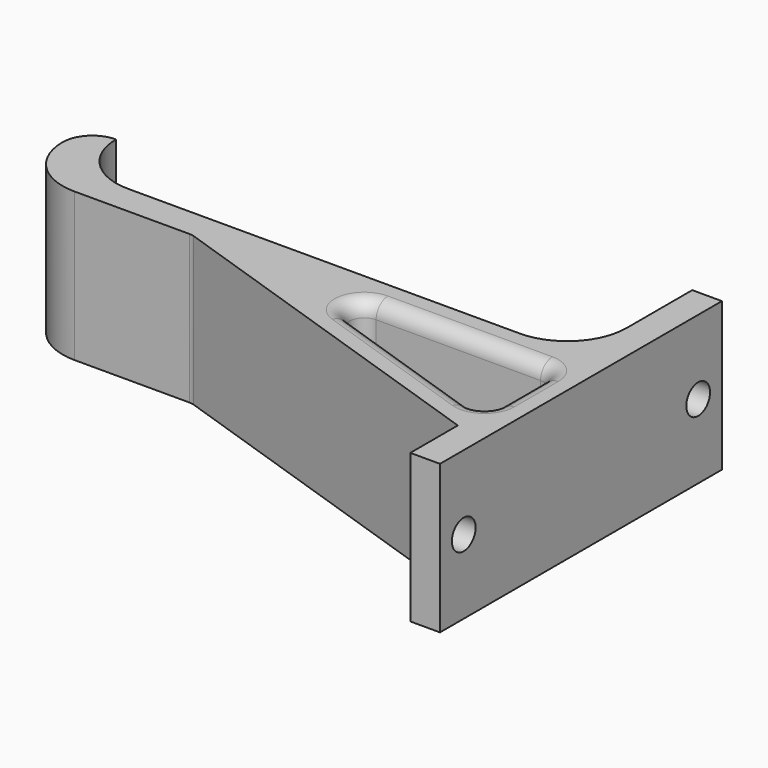
from build123d import *

# Parameters (mm, degrees)
F1_DEPTH = 25
F2_R     = 2.5
F3_DEPTH = 25
F4_R     = 4.99999
F5_F1_R  = 2.5
F5_F2_R  = 2.5
F5_F3_R  = 2.5


# Not quite as in the source:
# - a fillet or chamfer is up to 0.001 mm smaller than in the source, because OpenCascade refuses the exact size
# - a feature names something its author has since deleted; it is built from what else it names


with BuildPart() as f1:
    # F0 (on Top) → F1 (new body)
    with BuildSketch(Plane.XY):
        with BuildLine():
            ThreePointArc((11.9032669473, 15), (8.9743347592, 7.9289321881), (1.9032669473, 5))
            Line((1.9032669473, 5), (-64.0967330527, 5))
            ThreePointArc((-64.0967330527, 5), (-71.1678008646, 7.9289321881), (-74.0967330527, 15))
            Line((-74.0967330527, 15), (-79.0967330527, 15))
            Line((-79.0967330527, 15), (-79.0967330527, 10))
            ThreePointArc((-79.0967330527, 10), (-76.1678008646, 2.9289321881), (-69.0967330527, 0))
            Line((-69.0967330527, 0), (-49.3079621117, 0))
            Line((-49.3079621117, 0), (11.9032669473, -20.5484238273))
            Line((11.9032669473, -20.5484238273), (11.9032669473, -30.5484238273))
            Line((11.9032669473, -30.5484238273), (16.9032669473, -30.5484238273))
            Line((16.9032669473, -30.5484238273), (16.9032669473, 15))
            Line((16.9032669473, 15), (16.9032669473, 28.8165863603))
            Line((16.9032669473, 28.8165863603), (11.9032669473, 28.8165863603))
            Line((11.9032669473, 28.8165863603), (11.9032669473, 15))
        make_face()
        Polygon((-33.5967330527, 0), (11.9032669473, 0), (11.9032669473, -15.2742119136), align=None, mode=Mode.SUBTRACT)
    extrude(amount=F1_DEPTH)

    # F2 (on face) → F3 (cut)
    with BuildSketch(Plane.YZ.offset(16.9032669473)):
        with Locations((-25.5484238273, 12.5)):
            Circle(F2_R)
        with Locations((23.8165863603, 12.5)):
            Circle(F2_R)
    extrude(amount=-F3_DEPTH, mode=Mode.SUBTRACT)

    # F4 (radius 5 in the source; OpenCascade refuses exactly that, so slightly less here)
    f4_edges = [f1.edges().sort_by_distance(p)[0] for p in [
        (-79.096733, 15, 12.5),
    ]]
    fillet(f4_edges, radius=F4_R)

    # F5: fillet of radius 2.5 on 10 edges, made by hand

    # F5_f1
    f5_f1_edges = [f1.edges().sort_by_distance(p)[0] for p in [
        (-33.5967330527, 0, 12.5),
        (11.9032669473, 0, 12.5),
        (11.9032669473, -15.2742119136, 12.5),
        (-49.3079621117, 0, 12.5),
    ]]
    fillet(f5_f1_edges, radius=F5_F1_R)

    # F5_f2
    f5_f2_edges = [f1.edges().sort_by_distance(p)[0] for p in [
        (8.9743347592, 7.9289321881, 0),
        (-71.1678008646, 7.9289321881, 0),
        (-31.0967330527, 5, 0),
        (11.9032669473, 21.9082931802, 0),
    ]]
    fillet(f5_f2_edges, radius=F5_F2_R)

    # F5_f3
    f5_f3_edges = [f1.edges().sort_by_distance(p)[0] for p in [
        (11.9032669473, -7.148931772, 25),
        (-4.4453294203, 0, 25),
        (-20.7612174023, -2.0969217328, 25),
        (11.1710339003, -0.732233047, 25),
        (10.8628862029, -13.8275215518, 25),
    ]]
    fillet(f5_f3_edges, radius=F5_F3_R)


solid = f1.part
